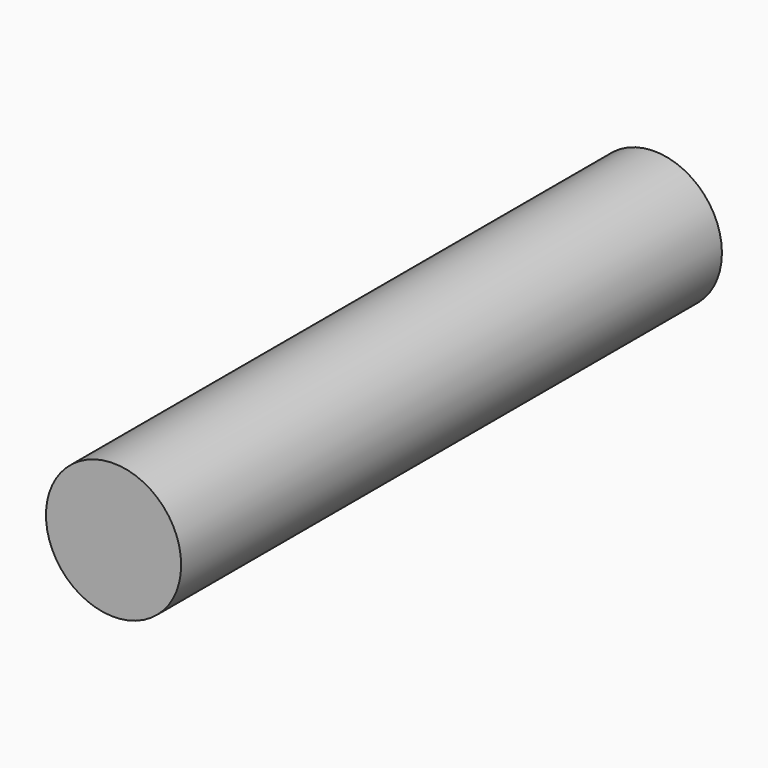
from build123d import *

# Parameters (mm, degrees)
F0_R     = 12.7
F1_DEPTH = 127


# Not quite as in the source:
# - a feature of the source that left no trace in its solid (it failed there, or was rolled back) is left out


with BuildPart() as f1:
    # F0 (on Front) → F1 (new body)
    with BuildSketch(Plane.XZ):
        Circle(F0_R)
    extrude(amount=F1_DEPTH)


solid = f1.part
